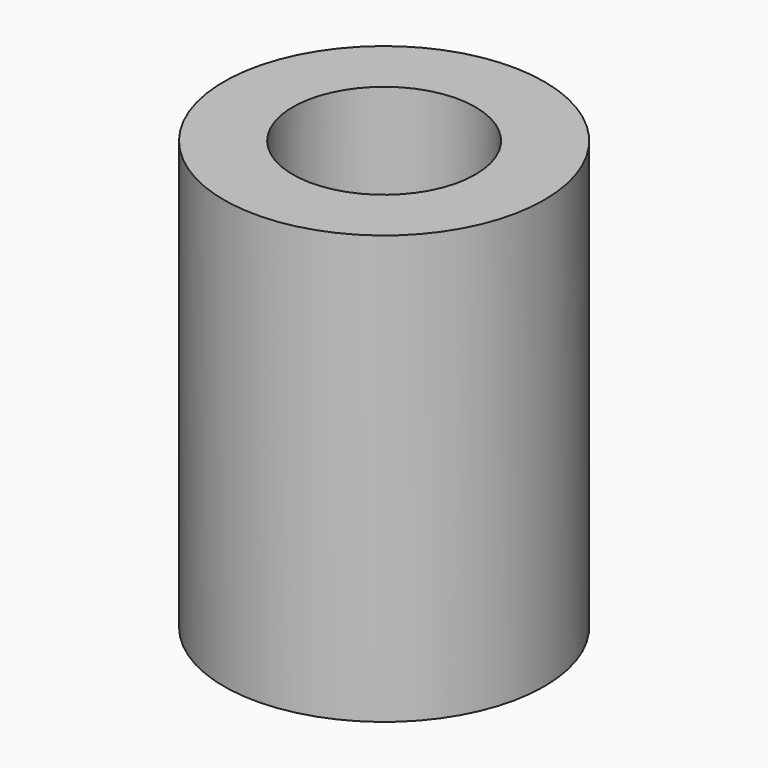
from build123d import *

# Parameters (mm, degrees)
F0_R     = 5.6107997284
F0_R_2   = 3.2
F1_DEPTH = 15


# Not quite as in the source:
# - a feature names something its author has since deleted; it is built from what else it names


with BuildPart() as f1:
    # F0 (on Top) → F1 (new body)
    with BuildSketch(Plane.XY):
        Circle(F0_R)
        Circle(F0_R_2, mode=Mode.SUBTRACT)
    extrude(amount=F1_DEPTH)


solid = f1.part
